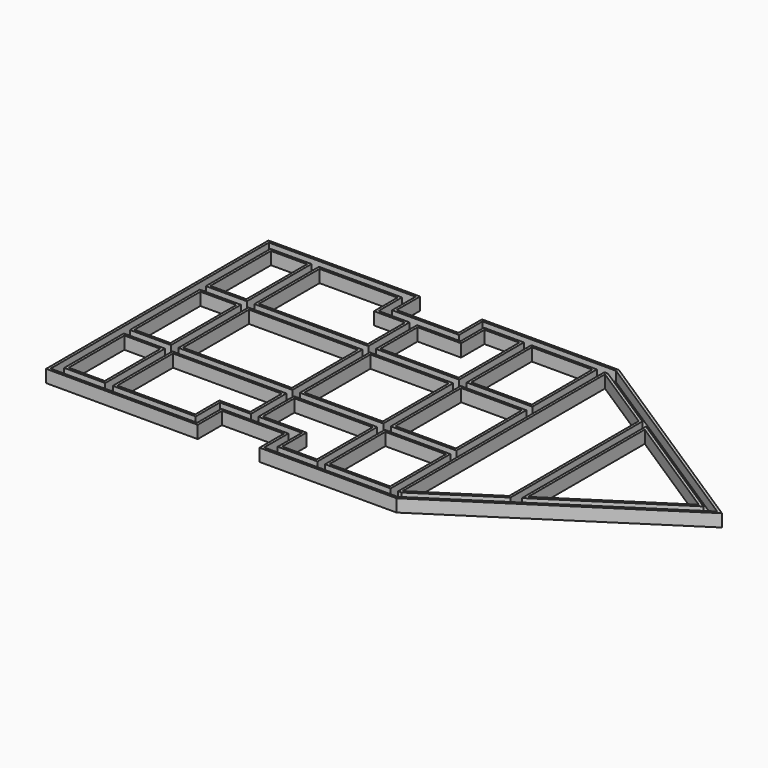
from build123d import *

# Parameters (mm, degrees)
F0_W     = 7.26223737
F0_H     = 14.0403658152
F0_H_2   = 16.6169349104
F0_W_2   = 21.9669826329
F0_W_3   = 15.7987792045
F0_W_4   = 12.2116522557
F0_H_3   = 15.2750127017
F1_DEPTH = 2.54
F2_T     = -0.508


with BuildPart() as f1:
    # F0 (on Top) → F1 (new body)
    with BuildSketch(Plane.XY):
        Polygon((-48.5124173612, 7.03542912), (-20.8847596319, 7.03542912), (22.3510192425, 35.0815849379), (-20.8847596319, 63.1277407557), (-48.5124173612, 63.1277407557), (-48.5124173612, 57.2236290348), (-60.9962199777, 57.2236290348), (-60.9962199777, 63.1277407557), (-91.6035394222, 63.1277407557), (-91.6035394222, 7.03542912), (-60.9962199777, 7.03542912), (-60.9962199777, 13.134556353), (-48.5124173612, 13.134556353), align=None)
        with Locations((-85.432421416, 16.5956113487)):
            Rectangle(F0_W, F0_H, mode=Mode.SUBTRACT)
        Polygon((-57.2943203151, 15.6745556742), (-63.5362192988, 15.6745556742), (-63.5362192988, 9.5754284412), (-79.261302948, 9.5754284412), (-79.261302948, 23.6157942563), (-57.2943203151, 23.6157942563), align=None, mode=Mode.SUBTRACT)
        Polygon((-38.955539465, 9.5754284412), (-45.97241804, 9.5754284412), (-45.97241804, 15.6745556742), (-54.7543186694, 15.6745556742), (-54.7543186694, 23.6157942563), (-38.955539465, 23.6157942563), align=None, mode=Mode.SUBTRACT)
        with Locations((-85.432421416, 34.4642614946)):
            Rectangle(F0_W, F0_H_2, mode=Mode.SUBTRACT)
        with Locations((-68.2778116316, 34.4642614946)):
            Rectangle(F0_W_2, F0_H_2, mode=Mode.SUBTRACT)
        with Locations((-46.8549290672, 34.4642614946)):
            Rectangle(F0_W_3, F0_H_2, mode=Mode.SUBTRACT)
        with Locations((-30.3097135541, 16.5956113487)):
            Rectangle(F0_W_4, F0_H, mode=Mode.SUBTRACT)
        with Locations((-30.3097135541, 34.4642614946)):
            Rectangle(F0_W_4, F0_H_2, mode=Mode.SUBTRACT)
        Polygon((-7.5185770554, 18.7333902767), (-21.6364338994, 9.5754284412), (-21.6638874263, 9.5754284412), (-21.6638874263, 23.6157942563), (-21.6638874263, 26.1557940394), (-21.6638874263, 42.7727289498), (-21.6638874263, 45.3127287328), (-21.6638874263, 60.5877414346), (-21.6364338994, 60.5877414346), (-7.5185770554, 51.429779599), align=None, mode=Mode.SUBTRACT)
        with Locations((-85.432421416, 52.9502350837)):
            Rectangle(F0_W, F0_H_3, mode=Mode.SUBTRACT)
        Polygon((-79.261302948, 60.5877414346), (-63.5362192988, 60.5877414346), (-63.5362192988, 54.6836297136), (-57.2943203151, 54.6836297136), (-57.2943203151, 45.3127287328), (-79.261302948, 45.3127287328), align=None, mode=Mode.SUBTRACT)
        Polygon((-54.7543186694, 54.6836297136), (-45.97241804, 54.6836297136), (-45.97241804, 60.5877414346), (-38.955539465, 60.5877414346), (-38.955539465, 45.3127287328), (-54.7543186694, 45.3127287328), align=None, mode=Mode.SUBTRACT)
        Polygon((-4.9785770554, 49.7821341158), (17.6836978644, 35.0815849379), (-4.9785770554, 20.38103576), align=None, mode=Mode.SUBTRACT)
        with Locations((-30.3097135541, 52.9502350837)):
            Rectangle(F0_W_4, F0_H_3, mode=Mode.SUBTRACT)
    extrude(amount=F1_DEPTH)

    # F2
    f2_openings = [f1.faces().sort_by_distance(p)[0] for p in [
        (-90.333422, 35.081585, 2.54),
    ]]
    offset(amount=F2_T, openings=f2_openings, kind=Kind.INTERSECTION)


solid = f1.part
